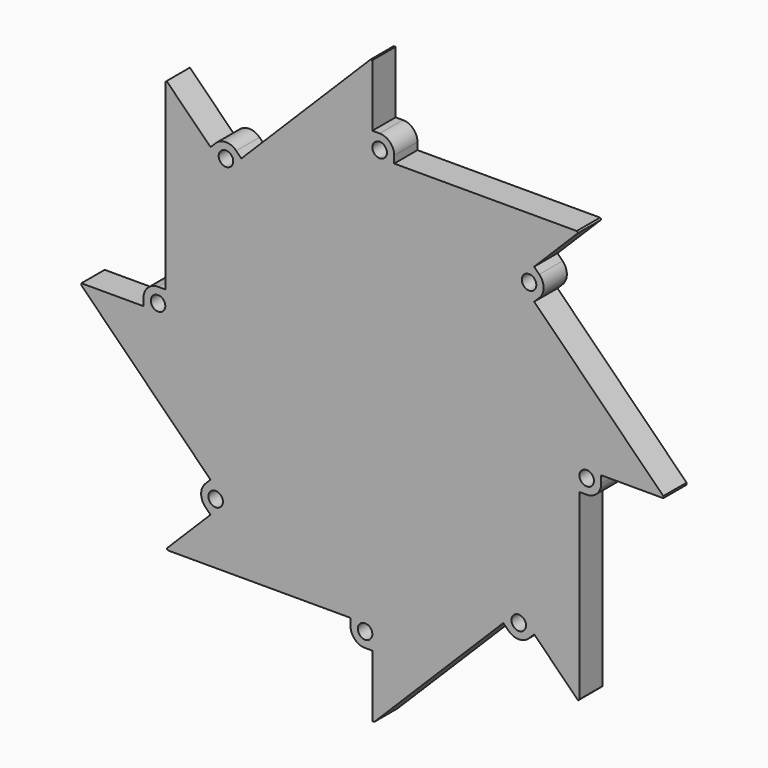
from build123d import *

# Parameters (mm, degrees)
F0_R            = 60
F2_DEPTH        = 6
F4_D            = 3
F4_COPIES_COUNT = 8
F6_DEPTH        = 25
F6_COPIES_COUNT = 8


# Not quite as in the source:
# - a pattern or mirror of a feature is missing from the dataset's text; its kind, count and spacing are read off the source's solid


with BuildPart() as f2:
    # F0 (on Front) → F2 (new body)
    with BuildSketch(Plane.XZ):
        Circle(F0_R)
    extrude(amount=F2_DEPTH)

    # F4 (through all)
    with Locations(Plane.XZ.offset(6)):
        with Locations((1.5, 44.1936596632)):
            f4 = Hole(F4_D / 2)

    # F4_copies: F4 ×8 about axis
    f4_copies_axis = Axis((0, 0, 0), (0, 1, 0))
    for i in range(1, F4_COPIES_COUNT):
        add(f4.rotate(f4_copies_axis, i * 360 / F4_COPIES_COUNT), mode=Mode.SUBTRACT)

    # F5 (on face) → F6 (cut)
    with BuildSketch(Plane.XZ.offset(6)):
        with BuildLine():
            Line((4.5, 44.1936596632), (4.5, 42.7004098892))
            Line((4.5, 42.7004098892), (42.1506227154, 42.7004098892))
            ThreePointArc((42.1506227154, 42.7004098892), (22.7813016161, 55.5068671128), (0, 60))
            Line((0, 60), (0, 47.1936596632))
            Line((0, 47.1936596632), (1.5, 47.1936596632))
            ThreePointArc((1.5, 47.1936596632), (3.6213203436, 46.3149800068), (4.5, 44.1936596632))
        make_face()
        with BuildLine():
            ThreePointArc((0, 60), (22.7813016161, 55.5068671128), (42.1506227154, 42.7004098892))
            Line((42.1506227154, 42.7004098892), (58.9860603213, 42.7004098892))
            Line((58.9860603213, 42.7004098892), (58.9860603213, 64.2154142261))
            Line((58.9860603213, 64.2154142261), (0, 64.2154142261))
            Line((0, 64.2154142261), (0, 60))
        make_face()
    f6 = extrude(amount=-F6_DEPTH, mode=Mode.SUBTRACT)

    # F6_copies: F6 ×8 about axis
    f6_copies_axis = Axis((0, 0, 0), (0, 1, 0))
    for i in range(1, F6_COPIES_COUNT):
        add(f6.rotate(f6_copies_axis, i * 360 / F6_COPIES_COUNT), mode=Mode.SUBTRACT)


solid = f2.part
